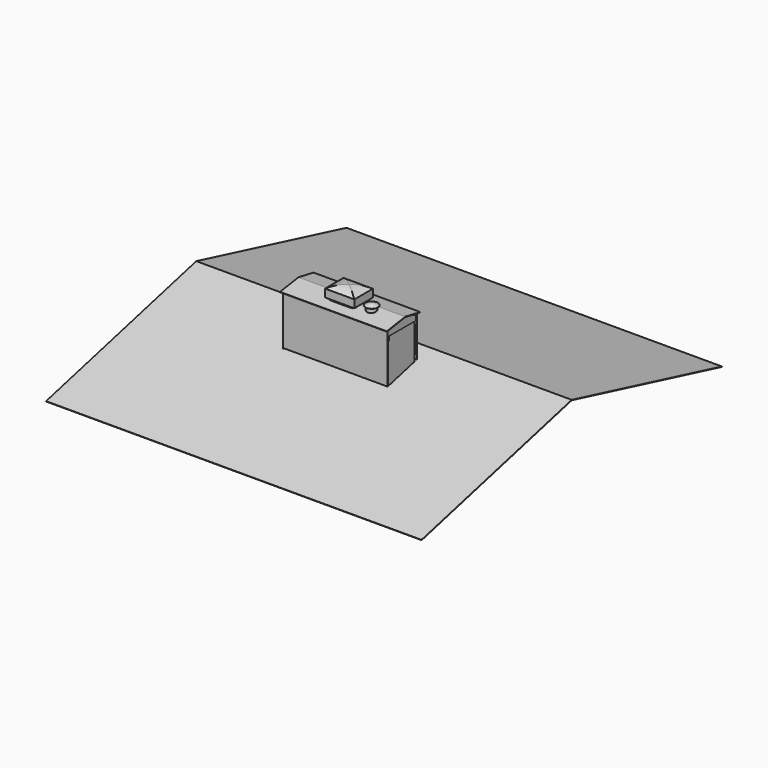
from build123d import *

# Parameters (mm, degrees)
F1_DEPTH       = 3048
F1_DEPTH_BACK  = 3048
F2_W           = 1657.35
F2_H           = 549.275
F3_DEPTH       = 762.001
F4_DEPTH       = 1270
F5_W           = 1682.75
F5_H           = 574.675
F6_DEPTH       = 76.2
F8_DEPTH       = 114.3
F7_R           = 76.2
F7_R_2         = 73.66
F9_DEPTH       = 1352.3614048759
F9_DEPTH_BACK  = 114.301
F11_DEPTH      = 1682.75
F12_DEPTH      = 114.3010001
F14_DEPTH      = 1466.6614048759
F15_W          = 476.25
F15_H          = 374.65
F16_DEPTH      = 101.6
F16_DEPTH_BACK = 25.4
F19_DEPTH      = 374.65
F20_DEPTH      = 3181.351
F21_DEPTH      = 127
F25_W          = 19.05
F25_H          = 63.5
F26_DEPTH      = 19.05
F25_W_2        = 44.45
F25_H_2        = 584.2
F27_DEPTH      = 19.05
F28_W          = 3.175
F28_H          = 63.5
F29_DEPTH      = 19.05
F30_DEPTH      = 19.05
F31_DEPTH      = 19.05
F32_DEPTH      = 19.05
F33_W          = 44.45
F33_H          = 406.4
F33_W_2        = 19.05
F34_DEPTH      = 19.05
F36_DEPTH      = 25.4
F36_DEPTH_BACK = 1708.15
F37_DEPTH      = 25.4
F37_DEPTH_BACK = 1708.15
F38_W          = 1694.5370192528
F38_H          = 108.1718015671
F38_H_2        = 63.5
F38_H_3        = 641.3647594452
F39_DEPTH      = 6.35
F40_W          = 552.45
F40_H          = 63.5
F41_DEPTH      = 6.35
F42_W          = 63.5
F42_H          = 406.4
F43_DEPTH      = 6.35


with BuildPart() as f1:
    # F0 (on Right) → F1 (new body, two sides)
    with BuildSketch(Plane.YZ) as f1_sk:
        Polygon((0, 762), (-3048, 0), (-3046.459898781, -6.1604048759), (0, 755.4545698193), (3046.459898781, -6.1604048759), (3048, 0), align=None)
    extrude(amount=F1_DEPTH)
    extrude(f1_sk.sketch, amount=-F1_DEPTH_BACK)

    # F2 (on Top) → F3 (cut, through all)
    with BuildSketch(Plane.XY):
        with Locations((-85.725, -579.4375)):
            Rectangle(F2_W, F2_H)
    extrude(amount=F3_DEPTH, mode=Mode.SUBTRACT)


with BuildPart() as f4:
    # F2 (on Top) → F4 (new body)
    with BuildSketch(Plane.XY):
        with Locations((-85.725, -579.4375)):
            Rectangle(F2_W, F2_H)
    extrude(amount=F4_DEPTH)

    # F5 (on face) → F6 (join)
    with BuildSketch(Plane.XY.offset(1270)):
        with Locations((-85.725, -579.4375)):
            Rectangle(F5_W, F5_H)
    extrude(amount=F6_DEPTH)

    # F7 (on face) → F8 (join)
    with BuildSketch(Plane.XY.offset(1346.2)):
        with BuildLine():
            Line((57.15, -419.1), (-266.7, -419.1))
            ThreePointArc((-266.7, -419.1), (-302.6210244843, -433.9789755157), (-317.5, -469.9))
            Line((-317.5, -469.9), (-317.5, -692.15))
            ThreePointArc((-317.5, -692.15), (-302.6210244843, -728.0710244843), (-266.7, -742.95))
            Line((-266.7, -742.95), (57.15, -742.95))
            ThreePointArc((57.15, -742.95), (93.0710244843, -728.0710244843), (107.95, -692.15))
            Line((107.95, -692.15), (107.95, -469.9))
            ThreePointArc((107.95, -469.9), (93.0710244843, -433.9789755157), (57.15, -419.1))
        make_face()
        with BuildLine():
            ThreePointArc((-285.75, -469.9), (-280.1703841816, -456.4296158184), (-266.7, -450.85))
            Line((-266.7, -450.85), (57.15, -450.85))
            ThreePointArc((57.15, -450.85), (70.6203841816, -456.4296158184), (76.2, -469.9))
            Line((76.2, -469.9), (76.2, -692.15))
            ThreePointArc((76.2, -692.15), (70.6203841816, -705.6203841816), (57.15, -711.2))
            Line((57.15, -711.2), (-266.7, -711.2))
            ThreePointArc((-266.7, -711.2), (-280.1703841816, -705.6203841816), (-285.75, -692.15))
            Line((-285.75, -692.15), (-285.75, -469.9))
        make_face(mode=Mode.SUBTRACT)
    extrude(amount=F8_DEPTH)

    # F7 (on face) → F9 (cut, two sides)
    with BuildSketch(Plane.XY.offset(1346.2)) as f9_sk:
        with Locations((311.15, -638.175)):
            Circle(F7_R)
        with Locations((311.15, -638.175)):
            Circle(F7_R_2, mode=Mode.SUBTRACT)
        with Locations((311.15, -638.175)):
            Circle(F7_R_2)
    extrude(amount=-F9_DEPTH, mode=Mode.SUBTRACT)
    extrude(f9_sk.sketch, amount=F9_DEPTH_BACK, mode=Mode.SUBTRACT)

    # F10 (on face) → F11 (join, through all)
    with BuildSketch(Plane.YZ.offset(755.65)):
        with BuildLine():
            Line((-866.775, 1346.2), (-292.1, 1346.2))
            ThreePointArc((-292.1, 1346.2), (-579.4375, 1416.05), (-866.775, 1346.2))
        make_face()
    extrude(amount=-F11_DEPTH)

    # F7 (on face) → F12 (cut, through all)
    with BuildSketch(Plane.XY.offset(1346.2)):
        with Locations((311.15, -638.175)):
            Circle(F7_R)
        with Locations((311.15, -638.175)):
            Circle(F7_R_2, mode=Mode.SUBTRACT)
        with Locations((311.15, -638.175)):
            Circle(F7_R_2)
    extrude(amount=F12_DEPTH, mode=Mode.SUBTRACT)

    # F13 (on face) → F14 (cut, through all)
    with BuildSketch(Plane.XY.offset(1460.5)):
        with BuildLine():
            Line((57.15, -450.85), (-266.7, -450.85))
            ThreePointArc((-266.7, -450.85), (-280.1703841816, -456.4296158184), (-285.75, -469.9))
            Line((-285.75, -469.9), (-285.75, -692.15))
            ThreePointArc((-285.75, -692.15), (-280.1703841816, -705.6203841816), (-266.7, -711.2))
            Line((-266.7, -711.2), (57.15, -711.2))
            ThreePointArc((57.15, -711.2), (70.6203841816, -705.6203841816), (76.2, -692.15))
            Line((76.2, -692.15), (76.2, -469.9))
            ThreePointArc((76.2, -469.9), (70.6203841816, -456.4296158184), (57.15, -450.85))
        make_face()
    extrude(amount=-F14_DEPTH, mode=Mode.SUBTRACT)

    # F33 (on face) → F34 (join)
    with BuildSketch(Plane(origin=(0, -304.8, 0), x_dir=(-1, 0, 0), z_dir=(0, 1, 0))):
        with Locations((-720.725, 1003.3)):
            Rectangle(F33_W, F33_H)
        with Locations((-752.475, 1003.3)):
            Rectangle(F33_W_2, F33_H)
    extrude(amount=F34_DEPTH)


with BuildPart() as f16:
    # F15 (on face) → F16 (new body, two sides)
    with BuildSketch(Plane.XY.offset(1460.5)) as f16_sk:
        with Locations((-104.775, -581.025)):
            Rectangle(F15_W, F15_H)
        Polygon((-266.7, -742.95), (-317.5, -742.95), (-317.5, -692.15), (-317.5, -469.9), (-317.5, -419.1), (-266.7, -419.1), (57.15, -419.1), (107.95, -419.1), (107.95, -469.9), (107.95, -692.15), (107.95, -742.95), (57.15, -742.95), align=None, mode=Mode.SUBTRACT)
    extrude(amount=F16_DEPTH)
    extrude(f16_sk.sketch, amount=-F16_DEPTH_BACK)

    # F17 (on face) → F19 (join, through all)
    with BuildSketch(Plane.XZ.offset(768.35)):
        with BuildLine():
            Line((-342.9, 1562.1), (133.35, 1562.1))
            ThreePointArc((133.35, 1562.1), (-104.775, 1625.6), (-342.9, 1562.1))
        make_face()
    extrude(amount=-F19_DEPTH)

    # F18 (on face) → F20 (cut, through all)
    with BuildSketch(Plane.YZ.offset(133.35)):
        with BuildLine():
            ThreePointArc((-768.35, 1562.1), (-581.025, 1625.6), (-393.7, 1562.1))
            Line((-393.7, 1562.1), (-393.7, 1738.6555246353))
            Line((-393.7, 1738.6555246353), (-768.35, 1738.6555246353))
            Line((-768.35, 1738.6555246353), (-768.35, 1562.1))
        make_face()
    extrude(amount=-F20_DEPTH, mode=Mode.SUBTRACT)


with BuildPart() as f21:
    # F7 (on face) → F21 (new body)
    with BuildSketch(Plane.XY.offset(1346.2)):
        with Locations((311.15, -638.175)):
            Circle(F7_R)
        with Locations((311.15, -638.175)):
            Circle(F7_R_2, mode=Mode.SUBTRACT)
    extrude(amount=F21_DEPTH)


with BuildPart() as f24:
    # F23 (on face) → F24 (revolve)
    with BuildSketch(Plane(origin=(311.15, 0, 0), x_dir=(0, -1, 0), z_dir=(-1, 0, 0))):
        Polygon((537.4668535416, 1483.521723889), (638.175, 1521.2872788109), (638.175, 1524), (536.575, 1485.9), align=None)
    revolve(axis=Axis((311.15, -638.175, 1497.3769187927), (0, 0, 1)))


with BuildPart() as f26:
    # F25 (on face) → F26 (new body)
    with BuildSketch(Plane.XZ.offset(854.075)):
        Polygon((742.95, 1270), (-914.4, 1270), (-914.4, 1206.5), (-869.95, 1206.5), (698.5, 1206.5), (742.95, 1206.5), align=None)
        with Locations((-923.925, 1238.25)):
            Rectangle(F25_W, F25_H)
        with Locations((752.475, 1238.25)):
            Rectangle(F25_W, F25_H)
    extrude(amount=F26_DEPTH)


with BuildPart() as f27:
    # F25 (on face) → F27 (new body)
    with BuildSketch(Plane.XZ.offset(854.075)):
        with Locations((-892.175, 914.4)):
            Rectangle(F25_W_2, F25_H_2)
        with Locations((-923.925, 914.4)):
            Rectangle(F25_W, F25_H_2)
    extrude(amount=F27_DEPTH)


with BuildPart() as f29:
    # F28 (on face) → F29 (new body)
    with BuildSketch(Plane(origin=(-914.4, 0, 0), x_dir=(0, -1, 0), z_dir=(-1, 0, 0))):
        Polygon((854.075, 1270), (304.8, 1270), (304.8, 1206.5), (365.125, 1206.5), (790.575, 1206.5), (854.075, 1206.5), align=None)
        with Locations((303.2125, 1238.25)):
            Rectangle(F28_W, F28_H)
    extrude(amount=F29_DEPTH)


with BuildPart() as f30:
    # F28 (on face) → F30 (new body)
    with BuildSketch(Plane(origin=(-914.4, 0, 0), x_dir=(0, -1, 0), z_dir=(-1, 0, 0))):
        Polygon((365.125, 1206.5), (304.8, 1206.5), (304.8, 757.9120133671), (365.125, 743.222006862), align=None)
        Polygon((304.8, 1206.5), (301.625, 1206.5), (301.625, 758.6851716042), (304.8, 757.9120133671), align=None)
    extrude(amount=F30_DEPTH)


with BuildPart() as f31:
    # F28 (on face) → F31 (new body)
    with BuildSketch(Plane(origin=(-914.4, 0, 0), x_dir=(0, -1, 0), z_dir=(-1, 0, 0))):
        Polygon((854.075, 624.1556383477), (854.075, 1206.5), (790.575, 1206.5), (790.575, 639.6188030899), align=None)
    extrude(amount=F31_DEPTH)


with BuildPart() as f32:
    # F28 (on face) → F32 (new body)
    with BuildSketch(Plane(origin=(-914.4, 0, 0), x_dir=(0, -1, 0), z_dir=(-1, 0, 0))):
        Polygon((365.125, 743.222006862), (304.8, 757.9120133671), (304.8, 692.5563750193), (854.075, 558.8), (854.075, 624.1556383477), (790.575, 639.6188030899), align=None)
        Polygon((304.8, 757.9120133671), (301.625, 758.6851716042), (301.625, 693.3295332564), (304.8, 692.5563750193), align=None)
    extrude(amount=F32_DEPTH)


with BuildPart() as f36:
    # F35 (on face) → F36 (new body, two sides)
    with BuildSketch(Plane(origin=(-927.1, 0, 0), x_dir=(0, -1, 0), z_dir=(-1, 0, 0))) as f36_sk:
        Polygon((546.1, 1434.8576312033), (546.1, 1428.4337425666), (674.0994462427, 1408.8504931516), (917.575, 1371.6), (918.535342417, 1377.8769612427), align=None)
    extrude(amount=F36_DEPTH)
    extrude(f36_sk.sketch, amount=-F36_DEPTH_BACK)


with BuildPart() as f37:
    # F35 (on face) → F37 (new body, two sides)
    with BuildSketch(Plane(origin=(-927.1, 0, 0), x_dir=(0, -1, 0), z_dir=(-1, 0, 0))) as f37_sk:
        Polygon((241.3, 1371.6), (546.1, 1428.4337425666), (546.1, 1434.8576312033), (240.1360254755, 1377.842408454), align=None)
    extrude(amount=F37_DEPTH)
    extrude(f37_sk.sketch, amount=-F37_DEPTH_BACK)


with BuildPart() as f39:
    # F38 (on face) → F39 (new body)
    with BuildSketch(Plane.XZ.offset(873.125)):
        with Locations((-85.2685096264, 1324.0859007835)):
            Rectangle(F38_W, F38_H)
        with Locations((-85.2685096264, 1238.25)):
            Rectangle(F38_W, F38_H_2)
        with Locations((-85.2685096264, 885.8176202774)):
            Rectangle(F38_W, F38_H_3)
    extrude(amount=F39_DEPTH)


with BuildPart() as f41:
    # F40 (on face) → F41 (new body)
    with BuildSketch(Plane(origin=(-933.45, 0, 0), x_dir=(0, -1, 0), z_dir=(-1, 0, 0))):
        Polygon((879.475, 1377.4291018017), (546.1, 1428.4337425666), (285.75, 1379.8882541243), (279.4, 1378.7042178208), (279.4, 698.7416409161), (285.75, 697.1953244419), (301.625, 693.3295332564), (854.075, 558.8), (879.475, 552.6147341032), (879.475, 565.1352405548), align=None)
        with Locations((577.85, 1238.25)):
            Rectangle(F40_W, F40_H, mode=Mode.SUBTRACT)
        with Locations((577.85, 1238.25)):
            Rectangle(F40_W, F40_H)
    extrude(amount=F41_DEPTH)


with BuildPart() as f43:
    # F42 (on face) → F43 (new body)
    with BuildSketch(Plane(origin=(0, -285.75, 0), x_dir=(-1, 0, 0), z_dir=(0, 1, 0))):
        Polygon((935.7254505157, 710.1965546608), (935.7254505157, 1380.3404569626), (-762, 1380.3404569626), (-762, 1206.5), (-698.5, 1206.5), (-698.5, 800.1), (-762, 800.1), (-762, 710.1965546608), align=None)
        with Locations((-730.25, 1003.3)):
            Rectangle(F42_W, F42_H)
    extrude(amount=F43_DEPTH)


solid = Compound([f1.part, f4.part, f16.part, f21.part, f24.part, f26.part, f27.part, f29.part, f30.part, f31.part, f32.part, f36.part, f37.part, f39.part, f41.part, f43.part])
